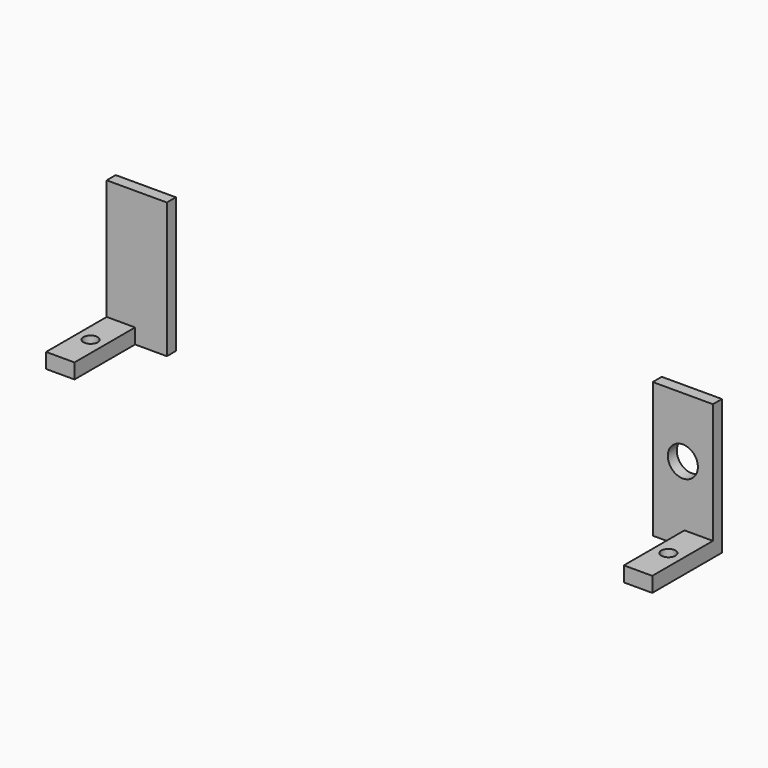
from build123d import *

# Parameters (mm, degrees)
F0_W     = 6
F0_H     = 16
F0_R     = 1.5
F1_DEPTH = 3.175
F2_DEPTH = 28.575
F3_R     = 3.175
F4_DEPTH = 2.38225


# Not quite as in the source:
# - a length typed as a fraction of an inch, garbled in the dataset ("3 / 203.2 mm" for 3/8 in), is restored


with BuildPart() as f1:
    # F0 (on Top) → F1 (new body)
    with BuildSketch(Plane.XY):
        with Locations((-61, 0)):
            Rectangle(F0_W, F0_H)
        with Locations((-61, 0)):
            Circle(F0_R, mode=Mode.SUBTRACT)
    extrude(amount=F1_DEPTH)

    # F0 (on Top) → F2, piece 2 (join)
    with BuildSketch(Plane.XY):
        Polygon((-64, 10.38125), (-64, 8), (-58, 8), (-51.3, 8), (-51.3, 10.38125), align=None)
    extrude(amount=F2_DEPTH)


with BuildPart() as f1b:
    # F0 (on Top) → F1, piece 2 (new body)
    with BuildSketch(Plane.XY):
        with Locations((61, 0)):
            Rectangle(F0_W, F0_H)
        with Locations((61, 0)):
            Circle(F0_R, mode=Mode.SUBTRACT)
    extrude(amount=F1_DEPTH)

    # F0 (on Top) → F2 (join)
    with BuildSketch(Plane.XY):
        Polygon((51.3, 8), (58, 8), (64, 8), (64, 10.38125), (51.3, 10.38125), align=None)
    extrude(amount=F2_DEPTH)

    # F3 (on face) → F4 (cut, through all)
    with BuildSketch(Plane.XZ.offset(-8)):
        with Locations((57.65, 15.875)):
            Circle(F3_R)
    extrude(amount=-F4_DEPTH, mode=Mode.SUBTRACT)


solid = Compound([f1.part, f1b.part])
